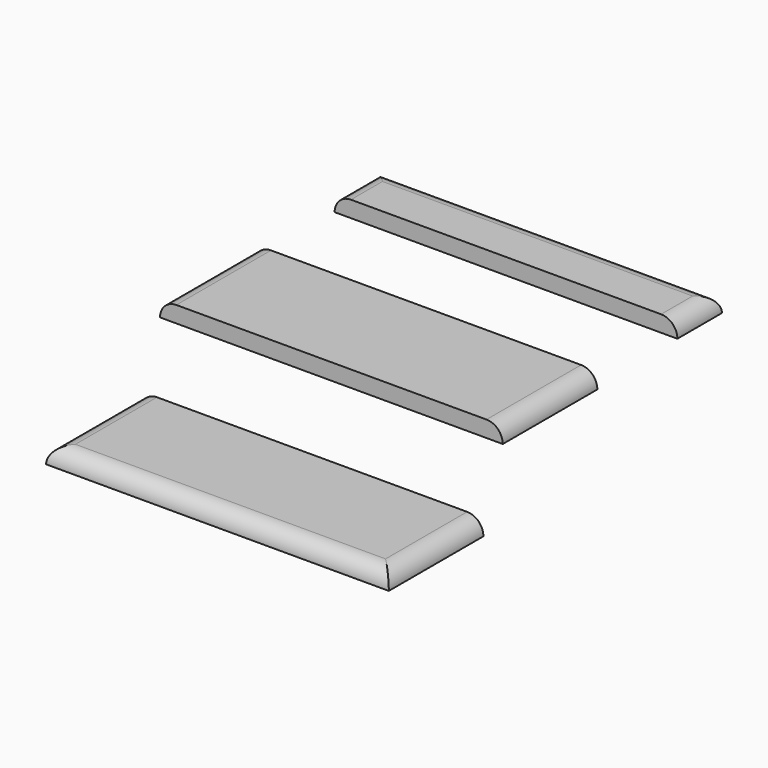
from build123d import *

# Parameters (mm, degrees)
F2_W     = 400
F2_H     = 65
F3_DEPTH = 19
F0_W     = 400
F0_H     = 138
F4_DEPTH = 19
F1_W     = 400
F1_H     = 138
F5_DEPTH = 19
F6_R     = 18.99999
F6_2_R   = 18.99999
F6_3_R   = 18.99999


# Not quite as in the source:
# - a fillet or chamfer is up to 0.001 mm smaller than in the source, because OpenCascade refuses the exact size


with BuildPart() as f3:
    # F2 (on Top) → F3 (new body)
    with BuildSketch(Plane.XY):
        with Locations((34.1459533652, 219.0565094352)):
            Rectangle(F2_W, F2_H)
    extrude(amount=F3_DEPTH)

    # F6#3 (radius 19 in the source; OpenCascade refuses exactly that, so slightly less here)
    f6_3_edges = [f3.edges().sort_by_distance(p)[0] for p in [
        (234.145953, 219.056509, 19),
        (34.145953, 251.556509, 19),
        (-165.854047, 219.056509, 19),
    ]]
    fillet(f6_3_edges, radius=F6_3_R)


with BuildPart() as f4:
    # F0 (on Top) → F4 (new body)
    with BuildSketch(Plane.XY):
        with Locations((39.6892666308, -6.0938838869)):
            Rectangle(F0_W, F0_H)
    extrude(amount=F4_DEPTH)

    # F6#2 (radius 19 in the source; OpenCascade refuses exactly that, so slightly less here)
    f6_2_edges = [f4.edges().sort_by_distance(p)[0] for p in [
        (-160.310733, -6.093884, 19),
        (239.689267, -6.093884, 19),
    ]]
    fillet(f6_2_edges, radius=F6_2_R)


with BuildPart() as f5:
    # F1 (on Top) → F5 (new body)
    with BuildSketch(Plane.XY):
        with Locations((139.6866820736, -297.3407134414)):
            Rectangle(F1_W, F1_H)
    extrude(amount=F5_DEPTH)

    # F6 (radius 19 in the source; OpenCascade refuses exactly that, so slightly less here)
    f6_edges = [f5.edges().sort_by_distance(p)[0] for p in [
        (139.686682, -366.340713, 19),
        (-60.313318, -297.340713, 19),
        (339.686682, -297.340713, 19),
    ]]
    fillet(f6_edges, radius=F6_R)


solid = Compound([f3.part, f4.part, f5.part])
